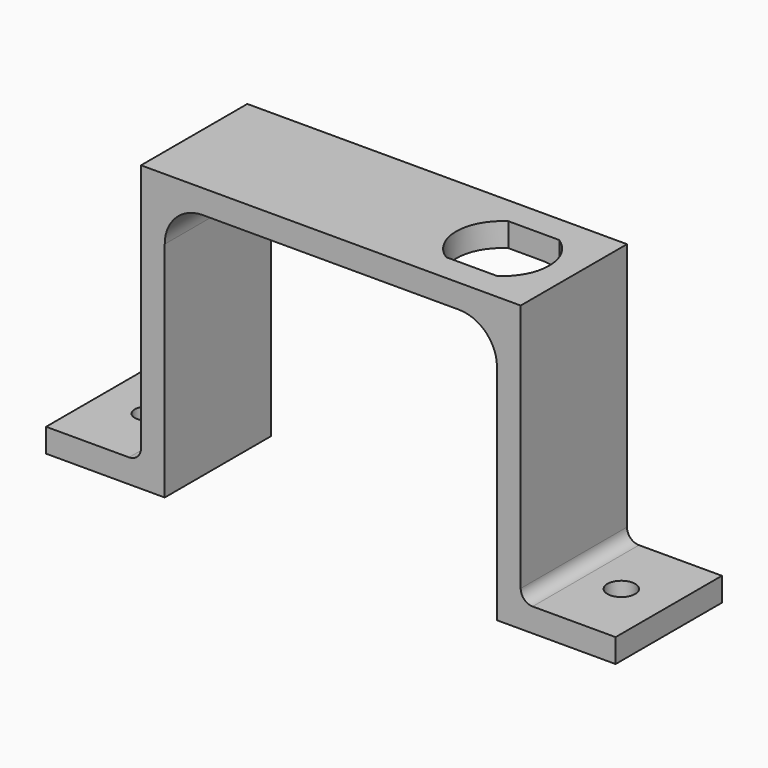
from build123d import *

# Parameters (mm, degrees)
F1_DEPTH     = 8.89
F2_R         = 1.5875
F2_R_2       = 1.8513271914
F3_DEPTH     = 3.176
F5_DEPTH     = 38.101
F6_T1_DEPTH  = 17.78
F6_T6_DEPTH  = 17.78
F6_S8_R      = 6.223
F6_T9_DEPTH  = 11
F6_T13_DEPTH = 17.78
F6_S16_R     = 6.223
F6_T17_DEPTH = 11
F6_T21_DEPTH = 17.78
F6_S23_R     = 6.223
F6_T24_DEPTH = 11
F6_T28_DEPTH = 17.78
F6_S30_R     = 6.223
F6_T31_DEPTH = 11
F6_T35_DEPTH = 17.78
F6_S37_R     = 6.223
F6_T38_DEPTH = 11
F7_R         = 1.6002


# Not quite as in the source:
# - a fillet or chamfer that OpenCascade refuses, or shapes differently, is made with other operations: its cross-section is extruded or revolved along the edge and cut away or added


with BuildPart() as f1:
    # F0 (on Front) → F1 (new body, symmetric)
    with BuildSketch(Plane.XZ):
        Polygon((-38.1, 3.175), (-38.1, 0), (-22.225, 0), (-22.225, 34.925), (22.225, 34.925), (22.225, 0), (38.1, 0), (38.1, 3.175), (25.4, 3.175), (25.4, 38.1), (-25.4, 38.1), (-25.4, 3.175), align=None)
    extrude(amount=F1_DEPTH, both=True)

    # F2 (on face) → F3 (cut, through all)
    with BuildSketch(Plane.XY.offset(3.175)):
        with Locations((-31.75, 0)):
            Circle(F2_R)
        with Locations((31.75, 0)):
            Circle(F2_R_2)
    extrude(amount=-F3_DEPTH, mode=Mode.SUBTRACT)

    # F4 (on face) → F5 (cut, through all)
    with BuildSketch(Plane.XY.offset(38.1)):
        with BuildLine():
            Line((19.2827675977, 5.207), (12.4672324023, 5.207))
            ThreePointArc((12.4672324023, 5.207), (9.652, 0), (12.4672324023, -5.207))
            Line((12.4672324023, -5.207), (19.2827675977, -5.207))
            ThreePointArc((19.2827675977, -5.207), (22.098, 0), (19.2827675977, 5.207))
        make_face()
    extrude(amount=-F5_DEPTH, mode=Mode.SUBTRACT)

    # F6: fillet of radius 5.08 on 2 edges, made by hand

    # F6_s2 → F6_t1 (join)
    with BuildSketch(Plane.XZ.offset(-8.89)):
        with BuildLine():
            ThreePointArc((-22.225, 29.845), (-20.7371024484, 33.4371024484), (-17.145, 34.925))
            Line((-17.145, 34.925), (-22.225, 34.925))
            Line((-22.225, 34.925), (-22.225, 29.845))
        make_face()
    extrude(amount=F6_T1_DEPTH)


with BuildPart() as f6_tool4:
    # F6_s5 → F6_t6 (new body)
    with BuildSketch(Plane.XZ.offset(-8.89)):
        with BuildLine():
            ThreePointArc((17.145, 34.925), (20.7371024484, 33.4371024484), (22.225, 29.845))
            Line((22.225, 29.845), (22.225, 34.925))
            Line((22.225, 34.925), (17.145, 34.925))
        make_face()
    extrude(amount=F6_T6_DEPTH)

    split(bisect_by=Plane.XZ.offset(-5.207), keep=Keep.BOTTOM)

    # F6_s8 → F6_t9 (cut, symmetric)
    with BuildSketch(Plane.XY.offset(32.4)):
        with Locations((15.875, 0)):
            Circle(F6_S8_R)
    extrude(amount=F6_T9_DEPTH, both=True, mode=Mode.SUBTRACT)


with BuildPart() as f1_1:
    add(f1.part)

    # F6_t3: union F6_tool4
    add(f6_tool4.part)


with BuildPart() as f6_tool11:
    # F6_s12 → F6_t13 (new body)
    with BuildSketch(Plane.XZ.offset(-8.89)):
        with BuildLine():
            ThreePointArc((17.145, 34.925), (20.7371024484, 33.4371024484), (22.225, 29.845))
            Line((22.225, 29.845), (22.225, 34.925))
            Line((22.225, 34.925), (17.145, 34.925))
        make_face()
    extrude(amount=F6_T13_DEPTH)

    split(bisect_by=Plane.XZ.offset(5.207), keep=Keep.BOTTOM)

    split(bisect_by=Plane.XZ.offset(-5.207), keep=Keep.TOP)

    # F6_s16 → F6_t17 (cut, symmetric)
    with BuildSketch(Plane.XY.offset(32.4)):
        with Locations((15.875, 0)):
            Circle(F6_S16_R)
    extrude(amount=F6_T17_DEPTH, both=True, mode=Mode.SUBTRACT)


with BuildPart() as f1_2:
    add(f1_1.part)

    # F6_t10: union F6_tool11
    add(f6_tool11.part)


with BuildPart() as f6_tool19:
    # F6_s20 → F6_t21 (new body)
    with BuildSketch(Plane.XZ.offset(-8.89)):
        with BuildLine():
            ThreePointArc((17.145, 34.925), (20.7371024484, 33.4371024484), (22.225, 29.845))
            Line((22.225, 29.845), (22.225, 34.925))
            Line((22.225, 34.925), (17.145, 34.925))
        make_face()
    extrude(amount=F6_T21_DEPTH)

    split(bisect_by=Plane.XZ.offset(-5.207), keep=Keep.BOTTOM)

    # F6_s23 → F6_t24 (intersect, symmetric)
    with BuildSketch(Plane.XY.offset(32.4)):
        with Locations((15.875, 0)):
            Circle(F6_S23_R)
    extrude(amount=F6_T24_DEPTH, both=True, mode=Mode.INTERSECT)


with BuildPart() as f1_3:
    add(f1_2.part)

    # F6_t18: union F6_tool19
    add(f6_tool19.part)


with BuildPart() as f6_tool26:
    # F6_s27 → F6_t28 (new body)
    with BuildSketch(Plane.XZ.offset(-8.89)):
        with BuildLine():
            ThreePointArc((17.145, 34.925), (20.7371024484, 33.4371024484), (22.225, 29.845))
            Line((22.225, 29.845), (22.225, 34.925))
            Line((22.225, 34.925), (17.145, 34.925))
        make_face()
    extrude(amount=F6_T28_DEPTH)

    split(bisect_by=Plane.XZ.offset(5.207), keep=Keep.TOP)

    # F6_s30 → F6_t31 (cut, symmetric)
    with BuildSketch(Plane.XY.offset(32.4)):
        with Locations((15.875, 0)):
            Circle(F6_S30_R)
    extrude(amount=F6_T31_DEPTH, both=True, mode=Mode.SUBTRACT)


with BuildPart() as f1_4:
    add(f1_3.part)

    # F6_t25: union F6_tool26
    add(f6_tool26.part)


with BuildPart() as f6_tool33:
    # F6_s34 → F6_t35 (new body)
    with BuildSketch(Plane.XZ.offset(-8.89)):
        with BuildLine():
            ThreePointArc((17.145, 34.925), (20.7371024484, 33.4371024484), (22.225, 29.845))
            Line((22.225, 29.845), (22.225, 34.925))
            Line((22.225, 34.925), (17.145, 34.925))
        make_face()
    extrude(amount=F6_T35_DEPTH)

    split(bisect_by=Plane.XZ.offset(5.207), keep=Keep.TOP)

    # F6_s37 → F6_t38 (intersect, symmetric)
    with BuildSketch(Plane.XY.offset(32.4)):
        with Locations((15.875, 0)):
            Circle(F6_S37_R)
    extrude(amount=F6_T38_DEPTH, both=True, mode=Mode.INTERSECT)


with BuildPart() as f1_5:
    add(f1_4.part)

    # F6_t32: union F6_tool33
    add(f6_tool33.part)

    # F7
    f7_edges = [f1_5.edges().sort_by_distance(p)[0] for p in [
        (-25.4, 0, 3.175),
        (25.4, 0, 3.175),
    ]]
    fillet(f7_edges, radius=F7_R)


solid = f1_5.part
